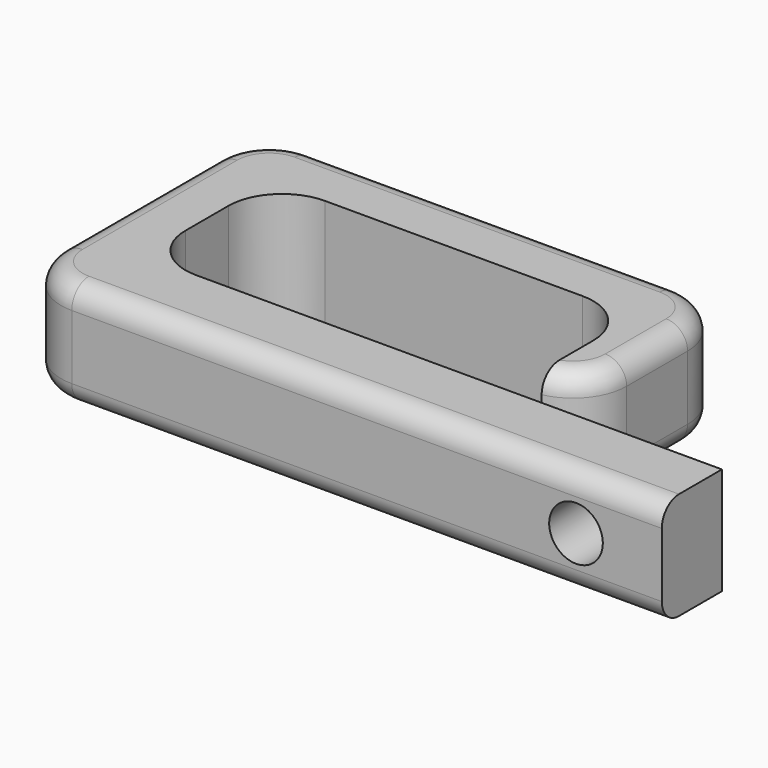
from build123d import *

# Parameters (mm, degrees)
F1_DEPTH       = 10
F3_D           = 5
F3_CBORE_D     = 9
F3_CBORE_DEPTH = 1.5
F4_T1_DEPTH    = 10
F4_T3_DEPTH    = 10
F4_T5_DEPTH    = 10
F4_T7_DEPTH    = 35
F4_T9_DEPTH    = 35
F4_T11_DEPTH   = 35
F4_T13_DEPTH   = 34.4948974279
F5_R           = 2


# Not quite as in the source:
# - a fillet or chamfer that OpenCascade refuses, or shapes differently, is made with other operations: its cross-section is extruded or revolved along the edge and cut away or added


with BuildPart() as f1:
    # F0 (on Top) → F1 (new body)
    with BuildSketch(Plane.XY):
        Polygon((-60, 0), (0, 0), (0, 7), (-54, 7), (-54, 22), (-20, 22), (-20, 11), (-16, 11), (-16, 28), (-60, 28), align=None)
    extrude(amount=F1_DEPTH)

    # F3 (through all)
    with Locations(Plane(origin=(0, 7, 0), x_dir=(-1, 0, 0), z_dir=(0, 1, 0))):
        with Locations((8, 5)):
            CounterBoreHole(F3_D / 2, F3_CBORE_D / 2, F3_CBORE_DEPTH)

    # F4: fillet of radius 5 on 7 edges, made by hand

    # F4_s2 → F4_t1 (join)
    with BuildSketch(Plane.XY):
        with BuildLine():
            ThreePointArc((-49, 7), (-52.5355339059, 8.4644660941), (-54, 12))
            Line((-54, 12), (-54, 7))
            Line((-54, 7), (-49, 7))
        make_face()
    extrude(amount=F4_T1_DEPTH)

    # F4_s4 → F4_t3 (join)
    with BuildSketch(Plane.XY):
        with BuildLine():
            ThreePointArc((-54, 17), (-52.5355339059, 20.5355339059), (-49, 22))
            Line((-49, 22), (-54, 22))
            Line((-54, 22), (-54, 17))
        make_face()
    extrude(amount=F4_T3_DEPTH)

    # F4_s6 → F4_t5 (join)
    with BuildSketch(Plane.XY):
        with BuildLine():
            ThreePointArc((-25, 22), (-21.4644660941, 20.5355339059), (-20, 17))
            Line((-20, 17), (-20, 22))
            Line((-20, 22), (-25, 22))
        make_face()
    extrude(amount=F4_T5_DEPTH)

    # F4_s8 → F4_t7 (cut)
    with BuildSketch(Plane.XY.offset(-12.5)):
        with BuildLine():
            ThreePointArc((-55, 0), (-58.5355339059, 1.4644660941), (-60, 5))
            Line((-60, 5), (-60, 0))
            Line((-60, 0), (-55, 0))
        make_face()
    extrude(amount=F4_T7_DEPTH, mode=Mode.SUBTRACT)

    # F4_s10 → F4_t9 (cut)
    with BuildSketch(Plane.XY.offset(-12.5)):
        with BuildLine():
            ThreePointArc((-60, 23), (-58.5355339059, 26.5355339059), (-55, 28))
            Line((-55, 28), (-60, 28))
            Line((-60, 28), (-60, 23))
        make_face()
    extrude(amount=F4_T9_DEPTH, mode=Mode.SUBTRACT)

    # F4_s12 → F4_t11 (cut)
    with BuildSketch(Plane.XY.offset(-12.5)):
        with BuildLine():
            ThreePointArc((-21, 28), (-17.4644660941, 26.5355339059), (-16, 23))
            Line((-16, 23), (-16, 28))
            Line((-16, 28), (-21, 28))
        make_face()
    extrude(amount=F4_T11_DEPTH, mode=Mode.SUBTRACT)

    # F4_s14 → F4_t13 (cut)
    with BuildSketch(Plane.XY.offset(-12.2474487139)):
        with BuildLine():
            ThreePointArc((-16, 15.8989794856), (-17.1270166538, 12.7367018254), (-20, 11))
            Line((-20, 11), (-16, 11))
            Line((-16, 11), (-16, 15.8989794856))
        make_face()
    extrude(amount=F4_T13_DEPTH, mode=Mode.SUBTRACT)

    # F5
    f5_edges = [f1.edges().sort_by_distance(p)[0] for p in [
        (-38, 28, 0),
        (-55, 28, 5),
        (-38, 28, 10),
        (-21, 28, 5),
        (-16, 19.44949, 0),
        (-16, 19.44949, 10),
        (-60, 14, 0),
        (-60, 14, 10),
        (-27.5, 0, 0),
        (-27.5, 0, 10),
        (-58.535534, 1.464466, 0),
        (-58.535534, 26.535534, 0),
        (-17.464466, 26.535534, 0),
        (-17.127017, 12.736702, 0),
        (-58.535534, 1.464466, 10),
        (-58.535534, 26.535534, 10),
        (-17.464466, 26.535534, 10),
        (-17.127017, 12.736702, 10),
    ]]
    fillet(f5_edges, radius=F5_R)


solid = f1.part
